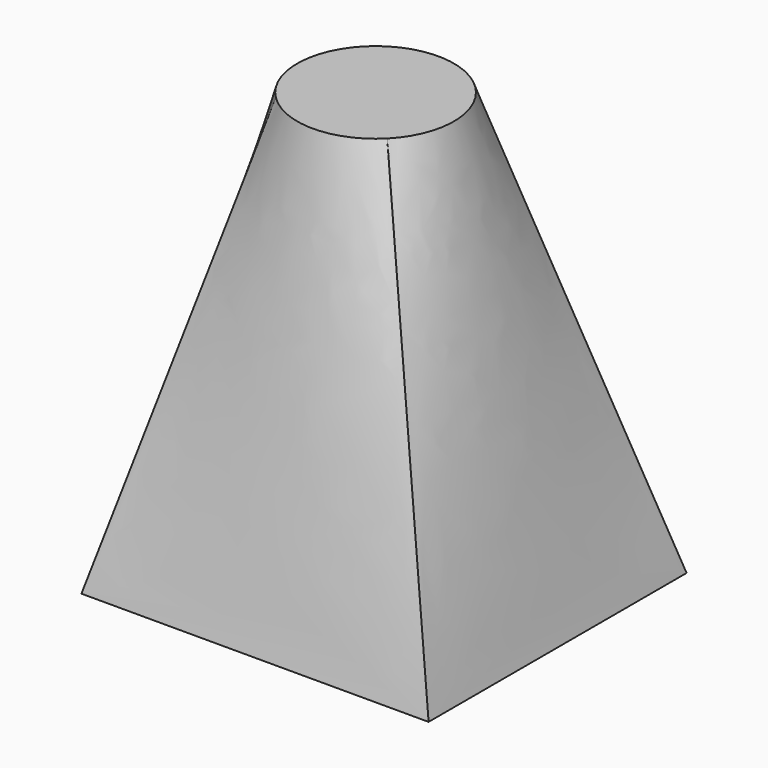
from build123d import *

# Parameters (mm, degrees)
F0_W = 65.6250044703
F0_H = 60.9621740878


# Not quite as in the source:
# - the arcs of a loft's sections are written as splines that run evenly, so that the points pair up as in the source's solid


with BuildPart() as f3:
    # F0 (on Top) → F3 section 0
    with BuildSketch(Plane.XY):
        with Locations((0, 1.986021176)):
            Rectangle(F0_W, F0_H)
    # F2 (on offset) → F3 section 1
    with BuildSketch(Plane.XY.offset(82.5)):
        with BuildLine():
            add(Edge.make_bspline(
                [(-10.5330555195, 10.4221814901), (-11.8973158864, 9.0434077468), (-12.9868922333, 7.3939150045), (-14.452448956, 3.8021136421), (-14.8278526978, 1.8612182422), (-14.8073276839, -2.0180177984), (-14.4114070039, -3.9548321255), (-12.9079250007, -7.5309243224), (-11.8009552334, -9.1687951527), (-10.4221814901, -10.5330555195)],
                knots=[0, 0, 0, 0, 0.25, 0.25, 0.5, 0.5, 0.75, 0.75, 1, 1, 1, 1], degree=3))
            add(Edge.make_bspline(
                [(-10.4221814901, -10.5330555195), (-9.0434077468, -11.8973158864), (-7.3939150045, -12.9868922333), (-3.8021136421, -14.452448956), (-1.8612182422, -14.8278526978), (2.0180177984, -14.8073276839), (3.9548321255, -14.4114070039), (7.5309243224, -12.9079250007), (9.1687951527, -11.8009552334), (10.5330555195, -10.4221814901)],
                knots=[0, 0, 0, 0, 0.25, 0.25, 0.5, 0.5, 0.75, 0.75, 1, 1, 1, 1], degree=3))
            add(Edge.make_bspline(
                [(10.5330555195, -10.4221814901), (11.8973158864, -9.0434077468), (12.9868922333, -7.3939150045), (14.452448956, -3.8021136421), (14.8278526978, -1.8612182422), (14.8073276839, 2.0180177984), (14.4114070039, 3.9548321255), (12.9079250007, 7.5309243224), (11.8009552334, 9.1687951527), (10.4221814901, 10.5330555195)],
                knots=[0, 0, 0, 0, 0.25, 0.25, 0.5, 0.5, 0.75, 0.75, 1, 1, 1, 1], degree=3))
            add(Edge.make_bspline(
                [(10.4221814901, 10.5330555195), (9.0434077468, 11.8973158864), (7.3939150045, 12.9868922333), (3.8021136421, 14.452448956), (1.8612182422, 14.8278526978), (-2.0180177984, 14.8073276839), (-3.9548321255, 14.4114070039), (-7.5309243224, 12.9079250007), (-9.1687951527, 11.8009552334), (-10.5330555195, 10.4221814901)],
                knots=[0, 0, 0, 0, 0.25, 0.25, 0.5, 0.5, 0.75, 0.75, 1, 1, 1, 1], degree=3))
        make_face()
    loft(ruled=True)


solid = f3.part
